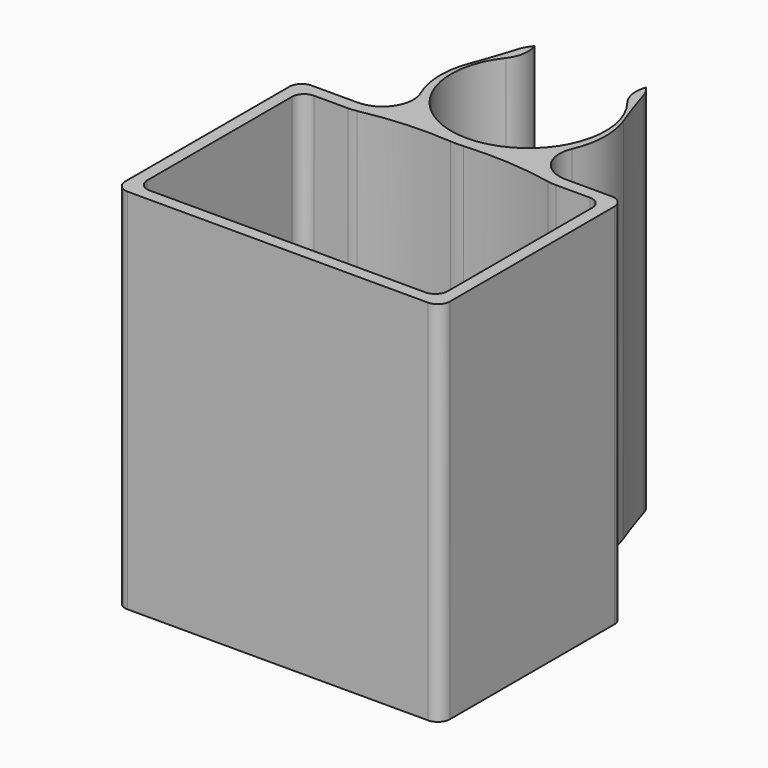
from build123d import *

# Parameters (mm, degrees)
F4_W        = 53
F4_H        = 35.5
F5_DEPTH    = 60
F6_T1_DEPTH = 60
F7_R        = 5.04
F9_T1_DEPTH = 74.3591672048
F10_T       = -2
F12_R       = 53
F13_R       = 2
F11_W       = 35
F11_H       = 21
F14_DEPTH   = 2
F15_R       = 3


# Not quite as in the source:
# - a fillet or chamfer that OpenCascade refuses, or shapes differently, is made with other operations: its cross-section is extruded or revolved along the edge and cut away or added
# - two fillets or chamfers of one size are made in one step


with BuildPart() as f5:
    # F4 (on Top) → F5 (new body)
    with BuildSketch(Plane.XY):
        with BuildLine():
            Line((-26.5, 0), (-26.5, -2))
            Line((-26.5, -2), (26.5, -2))
            Line((26.5, -2), (26.5, 0))
            Line((26.5, 0), (5.0951280026, 0))
            ThreePointArc((5.0951280026, 0), (0, -1), (-5.0951280026, 0))
            Line((-5.0951280026, 0), (-26.5, 0))
        make_face()
        with Locations((0, -19.75)):
            Rectangle(F4_W, F4_H)
        with BuildLine():
            ThreePointArc((-9.414110408, 22.1284476932), (-13.2305158305, 9.8978613101), (-5.0951280026, 0))
            Line((-5.0951280026, 0), (5.0951280026, 0))
            ThreePointArc((5.0951280026, 0), (13.2305158305, 9.8978613101), (9.414110408, 22.1284476932))
            ThreePointArc((9.414110408, 22.1284476932), (8.753655045, 22.7314262234), (8.0546720819, 23.2892857143))
            ThreePointArc((8.0546720819, 23.2892857143), (0, 1), (-8.0546720819, 23.2892857143))
            ThreePointArc((-8.0546720819, 23.2892857143), (-8.753655045, 22.7314262234), (-9.414110408, 22.1284476932))
        make_face()
        with BuildLine():
            Line((5.0951280026, 0), (-5.0951280026, 0))
            ThreePointArc((-5.0951280026, 0), (0, -1), (5.0951280026, 0))
        make_face()
        with BuildLine():
            Line((-9.414110408, 27.0511904762), (-9.414110408, 22.1284476932))
            ThreePointArc((-9.414110408, 22.1284476932), (-8.753655045, 22.7314262234), (-8.0546720819, 23.2892857143))
            Line((-8.0546720819, 23.2892857143), (-9.414110408, 27.0511904762))
        make_face()
        with BuildLine():
            ThreePointArc((8.0546720819, 23.2892857143), (8.753655045, 22.7314262234), (9.414110408, 22.1284476932))
            Line((9.414110408, 22.1284476932), (9.414110408, 27.0511904762))
            Line((9.414110408, 27.0511904762), (8.0546720819, 23.2892857143))
        make_face()
    extrude(amount=F5_DEPTH)

    # F6: fillet of radius 126 on 2 edges, made by hand

    # F6_s2 → F6_t1 (join)
    with BuildSketch(Plane.XY):
        with BuildLine():
            ThreePointArc((-9.414110408, 27.0511904762), (-10.9216954082, 22.0848726308), (-12.632526933, 17.1848541647))
            ThreePointArc((-12.632526933, 17.1848541647), (-11.297049781, 19.8348574754), (-9.414110408, 22.1284476932))
            Line((-9.414110408, 22.1284476932), (-9.414110408, 27.0511904762))
        make_face()
        with BuildLine():
            ThreePointArc((12.632526933, 17.1848541647), (10.9216954082, 22.0848726308), (9.414110408, 27.0511904762))
            Line((9.414110408, 27.0511904762), (9.414110408, 22.1284476932))
            ThreePointArc((9.414110408, 22.1284476932), (11.297049781, 19.8348574754), (12.632526933, 17.1848541647))
        make_face()
    extrude(amount=F6_T1_DEPTH)

    # F7
    f7_edges = [f5.edges().sort_by_distance(p)[0] for p in [
        (-5.095128, 0, 30),
        (5.095128, 0, 30),
        (8.054672, 23.289286, 30),
        (-8.054672, 23.289286, 30),
    ]]
    fillet(f7_edges, radius=F7_R)

    # F9: fillet of radius 5.04 on 2 edges, made by hand

    # F9_s2 → F9_t1 (cut)
    with BuildSketch(Plane.XY.offset(-7.1795836024)):
        with BuildLine():
            ThreePointArc((10.2229827876, 24.2956228784), (9.778060574, 25.324045565), (9.116903363, 26.2287444879))
            Line((9.116903363, 26.2287444879), (9.414110408, 27.0511904762))
            ThreePointArc((9.414110408, 27.0511904762), (9.8106956175, 25.6711020918), (10.2229827876, 24.2956228784))
        make_face()
        with BuildLine():
            ThreePointArc((-10.2229827876, 24.2956228784), (-9.778060574, 25.324045565), (-9.116903363, 26.2287444879))
            Line((-9.116903363, 26.2287444879), (-9.414110408, 27.0511904762))
            ThreePointArc((-9.414110408, 27.0511904762), (-9.8106956175, 25.6711020918), (-10.2229827876, 24.2956228784))
        make_face()
    extrude(amount=F9_T1_DEPTH, mode=Mode.SUBTRACT)

    # F10
    f10_openings = [f5.faces().sort_by_distance(p)[0] for p in [
        (0, -17.249718, 60),
    ]]
    offset(amount=F10_T, openings=f10_openings)

    # F12
    f12_edges = [f5.edges().sort_by_distance(p)[0] for p in [
        (-10.182168, 3.136566, 31),
        (10.182168, 3.136566, 31),
    ]]
    fillet(f12_edges, radius=F12_R)

    # F13
    f13_edges = [f5.edges().sort_by_distance(p)[0] for p in [
        (-26.5, 0, 30),
        (26.5, 0, 30),
        (24.5, -35.5, 31),
        (-24.5, -35.5, 31),
        (26.5, -37.5, 30),
        (-26.5, -37.5, 30),
        (24.5, -2, 31),
        (-24.5, -2, 31),
    ]]
    fillet(f13_edges, radius=F13_R)

    # F11 (on face) → F14 (cut)
    with BuildSketch(Plane(origin=(0, 0, 0), x_dir=(1, 0, 0), z_dir=(0, 0, -1))):
        with Locations((0, 18.75)):
            Rectangle(F11_W, F11_H)
    extrude(amount=-F14_DEPTH, mode=Mode.SUBTRACT)

    # F15
    f15_edges = [f5.edges().sort_by_distance(p)[0] for p in [
        (17.5, -8.25, 1),
        (-17.5, -8.25, 1),
        (-17.5, -29.25, 1),
        (17.5, -29.25, 1),
    ]]
    fillet(f15_edges, radius=F15_R)


solid = f5.part
